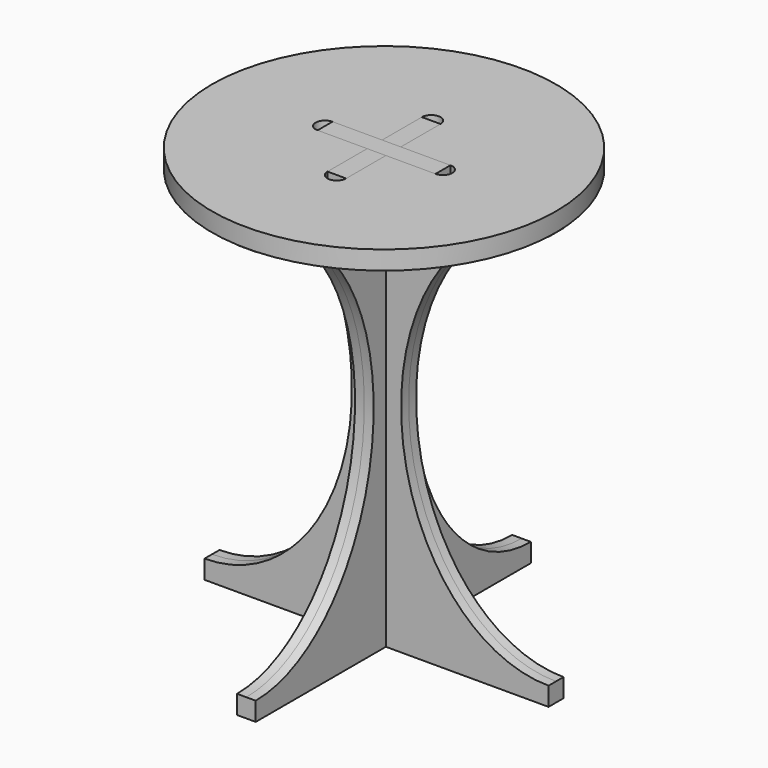
from build123d import *

# Parameters (mm, degrees)
F1_DEPTH      = 9.5
F1_DEPTH_BACK = 9.5
F5_R          = 175
F6_DEPTH      = 19
F7_W          = 120
F7_H          = 19
F8_DEPTH      = 440.0010001


# Not quite as in the source:
# - a feature of the source that left no trace in its solid (it failed there, or was rolled back) is left out
# - a pattern or mirror of a feature is missing from the dataset's text; its kind, count and spacing are read off the source's solid


with BuildPart() as f1:
    # F0 (on Front) → F1 (new body, two sides)
    with BuildSketch(Plane.XZ) as f1_sk:
        with BuildLine():
            Line((0, -220), (0, 220))
            Line((0, 220), (-60, 220))
            Line((-60, 220), (-60, 201))
            Line((-60, 201), (-175, 201))
            add(Edge.make_bspline(
                [(-175, -201), (-25, -201), (-25, 0), (-25, 201), (-175, 201)],
                knots=[0, 0, 0, 1.5707963268, 1.5707963268, 3.1415926536, 3.1415926536, 3.1415926536], degree=2, weights=[1, 0.7071067812, 1, 0.7071067812, 1]))
            Line((-175, -201), (-175, -220))
            Line((-175, -220), (0, -220))
        make_face()
    extrude(amount=F1_DEPTH)
    extrude(f1_sk.sketch, amount=-F1_DEPTH_BACK)


with BuildPart() as f1_copies_1:
    # F1_copies: instance of F1
    add(f1.part.mirror(Plane(origin=(0, 0, 0), x_dir=(0.7071067812, -0.7071067812, 0), z_dir=(0.7071067812, 0.7071067812, 0))))

    # F1_copies1: F1 across plane
    add(f1.part.mirror(Plane(origin=(0, 0, 0), x_dir=(-0.7071067812, -0.7071067812, 0), z_dir=(0.7071067812, -0.7071067812, 0))))


with BuildPart() as f1_1:
    add(f1.part)

    # F2: F1 across plane
    add(f1.part.mirror(Plane.YZ))


with BuildPart() as f6:
    # F5 (on face) → F6 (new body)
    with BuildSketch(Plane.XY.offset(220)):
        Circle(F5_R)
    extrude(amount=-F6_DEPTH)

    # F7 (on face) → F8 (cut, through all)
    with BuildSketch(Plane.XY.offset(220)):
        Rectangle(F7_W, F7_H)
        with BuildLine():
            ThreePointArc((-60, 9.5), (-69.5, 0), (-60, -9.5))
            Line((-60, -9.5), (-60, 9.5))
        make_face()
        with BuildLine():
            Line((60, 9.5), (60, -9.5))
            ThreePointArc((60, -9.5), (69.5, 0), (60, 9.5))
        make_face()
    f8 = extrude(amount=-F8_DEPTH, mode=Mode.SUBTRACT)

    # F8_copies: F8 across plane
    add(f8.mirror(Plane(origin=(0, 0, 0), x_dir=(0.7071067812, -0.7071067812, 0), z_dir=(-0.7071067812, -0.7071067812, 0))), mode=Mode.SUBTRACT)


solid = Compound([f1_copies_1.part, f1_1.part, f6.part])
